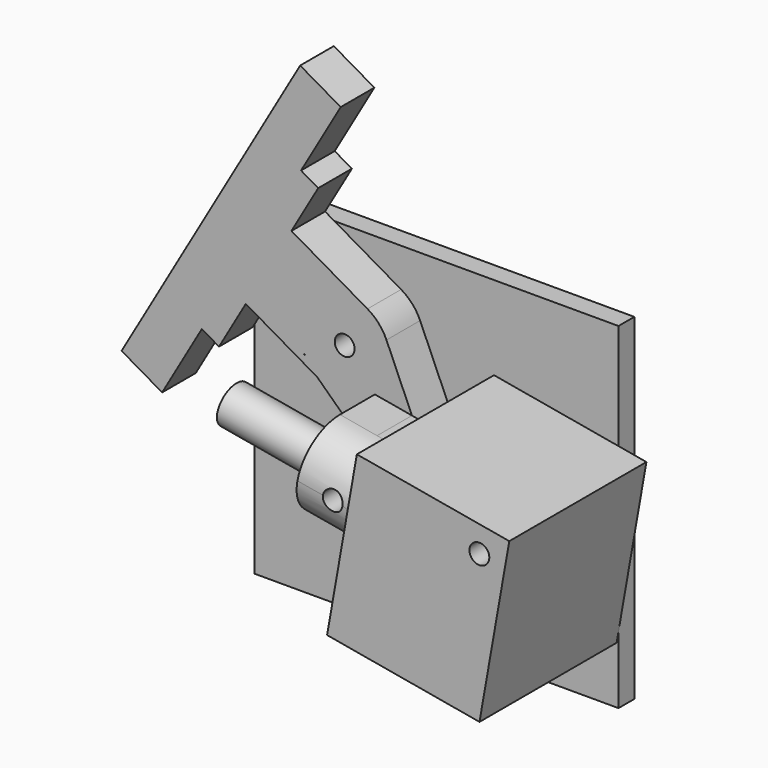
from build123d import *

# Parameters (mm, degrees)
F1_DEPTH    = 10.6
F2_DEPTH    = 43.2
F3_R        = 11
F4_DEPTH    = 2
F5_R        = 5
F6_DEPTH    = 43.4
F7_R        = 2.5
F8_DEPTH    = 22
F9_T1_DEPTH = 73
F9_T3_DEPTH = 73
F10_W       = 91.6676837951
F10_H       = 84.7782492638
F11_DEPTH   = 5
F12_R       = 2.5
F13_DEPTH   = 74.8
F15_DEPTH   = 10.6


# Not quite as in the source:
# - a fillet or chamfer that OpenCascade refuses, or shapes differently, is made with other operations: its cross-section is extruded or revolved along the edge and cut away or added
# - a feature of the source that left no trace in its solid (it failed there, or was rolled back) is left out
# - a feature names something its author has since deleted; it is built from what else it names


with BuildPart() as f1:
    # F0 (on Front) → F1 (new body)
    with BuildSketch(Plane.XZ):
        with BuildLine():
            Line((20.5230552312, -18.1992913043), (10.5343781692, 4.6126864827))
            ThreePointArc((10.5343781692, 4.6126864827), (0.6372216988, 11.4823320152), (-9.9592921435, 5.75))
            ThreePointArc((-9.9592921435, 5.75), (-11.496683076, 0.276185173), (-10.2239091523, -5.2651383312))
            Line((-10.2239091523, -5.2651383312), (-10.0330621935, -5.2987897992))
            Line((-10.0330621935, -5.2987897992), (-10.0760856471, -5.5427879295))
            ThreePointArc((-10.0760856471, -5.5427879295), (-9.1133059009, -7.0141040451), (-7.937476981, -8.3214457383))
            Line((-7.937476981, -8.3214457383), (0.0076867142, -15.9000031098))
            ThreePointArc((0.0076867142, -15.9000031098), (4.1721880916, -16.865197921), (7.4918654025, -19.5586001001))
            Line((7.4918654025, -19.5586001001), (12.1068221008, -20.3723414808))
            ThreePointArc((12.1068221008, -20.3723414808), (14.7867308402, -18.3159751797), (17.0688414833, -20.8064619249))
            ThreePointArc((17.0688414833, -20.8064619249), (17.0593282285, -21.0243512818), (17.0308608658, -21.2405823691))
            Line((17.0308608658, -21.2405823691), (20.9700918779, -21.9351750798))
            ThreePointArc((20.9700918779, -21.9351750798), (21.0227999926, -20.0341798777), (20.5230552312, -18.1992913043))
        make_face()
        with BuildLine():
            ThreePointArc((2.5, 0), (-0.6470476128, -2.4148145657), (-2.1650635095, 1.25))
            ThreePointArc((-2.1650635095, 1.25), (0.6470476128, 2.4148145657), (2.5, 0))
        make_face(mode=Mode.SUBTRACT)
        with BuildLine():
            ThreePointArc((10.0824414506, -25.509887777), (16.5964769767, -26.9821152755), (20.9700918779, -21.9351750798))
            Line((20.9700918779, -21.9351750798), (17.0308608658, -21.2405823691))
            ThreePointArc((17.0308608658, -21.2405823691), (14.1347210391, -23.2684813075), (12.1068221008, -20.3723414808))
            Line((12.1068221008, -20.3723414808), (7.4918654025, -19.5586001001))
            ThreePointArc((7.4918654025, -19.5586001001), (8.9071937501, -22.0966835606), (9.4890434601, -24.9438704))
            Line((9.4890434601, -24.9438704), (10.0824414506, -25.509887777))
        make_face()
        with BuildLine():
            Line((3.0158426859, -18.7693565289), (9.4890434601, -24.9438704))
            ThreePointArc((9.4890434601, -24.9438704), (8.9071937501, -22.0966835606), (7.4918654025, -19.5586001001))
            Line((7.4918654025, -19.5586001001), (3.0158426859, -18.7693565289))
        make_face()
        with BuildLine():
            ThreePointArc((7.4918654025, -19.5586001001), (4.1721880916, -16.865197921), (0.0076867142, -15.9000031098))
            Line((0.0076867142, -15.9000031098), (3.0158426859, -18.7693565289))
            Line((3.0158426859, -18.7693565289), (7.4918654025, -19.5586001001))
        make_face()
    extrude(amount=F1_DEPTH)

    # F14 (on face) → F15 (join)
    with BuildSketch(Plane.XZ.offset(10.6)):
        with BuildLine():
            Line((-31.664557856, -10.5859724576), (-24.914557856, 1.1053704935))
            Line((-24.914557856, 1.1053704935), (-6.941731015, -9.2712459212))
            Line((-6.941731015, -9.2712459212), (-7.937476981, -8.3214457383))
            ThreePointArc((-7.937476981, -8.3214457383), (-9.1133059009, -7.0141040451), (-10.0760856471, -5.5427879295))
            ThreePointArc((-10.0760856471, -5.5427879295), (-10.1509467311, -5.4044685642), (-10.2239091523, -5.2651383312))
            ThreePointArc((-10.2239091523, -5.2651383312), (-11.496683076, 0.276185173), (-9.9592921435, 5.75))
            Line((-9.9592921435, 5.75), (-23.4946848749, 13.564662637))
            Line((-23.4946848749, 13.564662637), (-35.9946848749, -8.0859724576))
            Line((-35.9946848749, -8.0859724576), (-31.664557856, -10.5859724576))
        make_face()
        with BuildLine():
            Line((-17.7446848749, 23.5239547806), (-23.4946848749, 13.564662637))
            Line((-23.4946848749, 13.564662637), (-9.9592921435, 5.75))
            ThreePointArc((-9.9592921435, 5.75), (-2.9764190187, 11.1081470023), (5.75, 9.9592921435))
            Line((5.75, 9.9592921435), (-13.414557856, 21.0239547806))
            Line((-13.414557856, 21.0239547806), (-6.664557856, 32.7152977317))
            Line((-6.664557856, 32.7152977317), (-10.9946848749, 35.2152977317))
            Line((-10.9946848749, 35.2152977317), (-17.7446848749, 23.5239547806))
        make_face()
        Polygon((-41.6238499995, -4.8359724576), (-35.9946848749, -8.0859724576), (-23.4946848749, 13.564662637), (-17.7446848749, 23.5239547806), (-10.9946848749, 35.2152977317), (-16.6238499995, 38.4652977317), align=None)
        Polygon((-45.9946848749, -25.4064805333), (-35.9946848749, -8.0859724576), (-41.6238499995, -4.8359724576), (-16.6238499995, 38.4652977317), (-10.9946848749, 35.2152977317), (-0.9946848749, 52.5358058073), (-11.2137846395, 58.4358058073), (-56.2137846395, -19.5064805333), align=None)
    extrude(amount=-F15_DEPTH)


with BuildPart() as f2:
    # F0 (on Front) → F2 (new body)
    with BuildSketch(Plane.XZ):
        Polygon((29.1525274041, -1.4447444142), (25.4017267665, -22.7165918793), (21.6509261288, -43.9884393443), (60.0584284963, -50.7607182734), (67.5600297715, -8.2170233432), align=None)
    extrude(amount=F2_DEPTH)

    # F3 (on face) → F4 (join)
    with BuildSketch(Plane(origin=(28.5205369873, 0, -5.0289401751), x_dir=(0, -1, 0), z_dir=(-0.984807753, 0, 0.1736481777))):
        with Locations((21.6, -17.9605122421)):
            Circle(F3_R)
    extrude(amount=F4_DEPTH)

    # F5 (on face) → F6 (join)
    with BuildSketch(Plane(origin=(26.5509214812, 0, -4.6816438198), x_dir=(0, -1, 0), z_dir=(-0.984807753, 0, 0.1736481777))):
        with Locations((21.6, -17.9605122421)):
            Circle(F5_R)
    extrude(amount=F6_DEPTH)


with BuildPart() as f8:
    # F7 (on face) → F8 (new body)
    with BuildSketch(Plane.XZ.offset(10.6)):
        with BuildLine():
            Line((3.7954417519, -30.0765136091), (21.5219813061, -33.2021808071))
            Line((21.5219813061, -33.2021808071), (25.3422412148, -11.5364102408))
            Line((25.3422412148, -11.5364102408), (16.9582685695, -10.0580896579))
            Line((16.9582685695, -10.0580896579), (20.5230552312, -18.1992913043))
            ThreePointArc((20.5230552312, -18.1992913043), (18.2970883196, -26.1309502128), (10.0824414506, -25.509887777))
            Line((10.0824414506, -25.509887777), (5.3899032629, -21.0338730293))
            Line((5.3899032629, -21.0338730293), (3.7954417519, -30.0765136091))
        make_face()
        with BuildLine():
            Line((20.5230552312, -18.1992913043), (16.9582685695, -10.0580896579))
            Line((16.9582685695, -10.0580896579), (7.6157016605, -8.4107430428))
            Line((7.6157016605, -8.4107430428), (5.3899032629, -21.0338730293))
            Line((5.3899032629, -21.0338730293), (10.0824414506, -25.509887777))
            ThreePointArc((10.0824414506, -25.509887777), (18.2970883196, -26.1309502128), (20.5230552312, -18.1992913043))
        make_face()
        with Locations((14.5688414833, -20.8064619249)):
            Circle(F7_R, mode=Mode.SUBTRACT)
    extrude(amount=F8_DEPTH)

    # F9: fillet of radius 11 on 2 edges, made by hand

    # F9_s2 → F9_t1 (cut)
    with BuildSketch(Plane(origin=(53.6331346891, 0, -9.4569687057), x_dir=(0, 1, 0), z_dir=(-0.984807753, 0, 0.1736481777))):
        with BuildLine():
            ThreePointArc((-21.6, 6.9605122421), (-29.3781745931, 10.1823376491), (-32.6, 17.9605122421))
            Line((-32.6, 17.9605122421), (-32.6, 6.9605122421))
            Line((-32.6, 6.9605122421), (-21.6, 6.9605122421))
        make_face()
    extrude(amount=F9_T1_DEPTH, mode=Mode.SUBTRACT)

    # F9_s4 → F9_t3 (cut)
    with BuildSketch(Plane(origin=(-18.2578312808, 0, 3.219348264), x_dir=(0, 1, 0), z_dir=(0.984807753, 0, -0.1736481777))):
        with BuildLine():
            ThreePointArc((-21.6, -28.9605122421), (-29.3781745931, -25.7386868352), (-32.6, -17.9605122421))
            Line((-32.6, -17.9605122421), (-32.6, -28.9605122421))
            Line((-32.6, -28.9605122421), (-21.6, -28.9605122421))
        make_face()
    extrude(amount=F9_T3_DEPTH, mode=Mode.SUBTRACT)


with BuildPart() as f11:
    # F10 (on face) → F11 (new body)
    with BuildSketch(Plane.XZ):
        with Locations((14.6878799424, -22.7255448699)):
            Rectangle(F10_W, F10_H)
        with BuildLine():
            Line((10.5343781692, 4.6126864827), (20.5230552312, -18.1992913043))
            ThreePointArc((20.5230552312, -18.1992913043), (21.0227999926, -20.0341798777), (20.9700918779, -21.9351750798))
            Line((20.9700918779, -21.9351750798), (17.0308608658, -21.2405823691))
            ThreePointArc((17.0308608658, -21.2405823691), (17.0593282285, -21.0243512818), (17.0688414833, -20.8064619249))
            ThreePointArc((17.0688414833, -20.8064619249), (14.7867308402, -18.3159751797), (12.1068221008, -20.3723414808))
            Line((12.1068221008, -20.3723414808), (7.4918654025, -19.5586001001))
            ThreePointArc((7.4918654025, -19.5586001001), (4.1721880916, -16.865197921), (0.0076867142, -15.9000031098))
            Line((0.0076867142, -15.9000031098), (-7.937476981, -8.3214457383))
            ThreePointArc((-7.937476981, -8.3214457383), (-9.1133059009, -7.0141040451), (-10.0760856471, -5.5427879295))
            Line((-10.0760856471, -5.5427879295), (-10.0330621935, -5.2987897992))
            Line((-10.0330621935, -5.2987897992), (-10.2239091523, -5.2651383312))
            ThreePointArc((-10.2239091523, -5.2651383312), (-11.496683076, 0.276185173), (-9.9592921435, 5.75))
            ThreePointArc((-9.9592921435, 5.75), (0.6372216988, 11.4823320152), (10.5343781692, 4.6126864827))
        make_face(mode=Mode.SUBTRACT)
    extrude(amount=-F11_DEPTH)

    # F0 (on Front) → F11, piece 2 (join)
    with BuildSketch(Plane.XZ):
        with BuildLine():
            Line((20.5230552312, -18.1992913043), (10.5343781692, 4.6126864827))
            ThreePointArc((10.5343781692, 4.6126864827), (0.6372216988, 11.4823320152), (-9.9592921435, 5.75))
            ThreePointArc((-9.9592921435, 5.75), (-11.496683076, 0.276185173), (-10.2239091523, -5.2651383312))
            Line((-10.2239091523, -5.2651383312), (-10.0330621935, -5.2987897992))
            Line((-10.0330621935, -5.2987897992), (-10.0760856471, -5.5427879295))
            ThreePointArc((-10.0760856471, -5.5427879295), (-9.1133059009, -7.0141040451), (-7.937476981, -8.3214457383))
            Line((-7.937476981, -8.3214457383), (0.0076867142, -15.9000031098))
            ThreePointArc((0.0076867142, -15.9000031098), (4.1721880916, -16.865197921), (7.4918654025, -19.5586001001))
            Line((7.4918654025, -19.5586001001), (12.1068221008, -20.3723414808))
            ThreePointArc((12.1068221008, -20.3723414808), (14.7867308402, -18.3159751797), (17.0688414833, -20.8064619249))
            ThreePointArc((17.0688414833, -20.8064619249), (17.0593282285, -21.0243512818), (17.0308608658, -21.2405823691))
            Line((17.0308608658, -21.2405823691), (20.9700918779, -21.9351750798))
            ThreePointArc((20.9700918779, -21.9351750798), (21.0227999926, -20.0341798777), (20.5230552312, -18.1992913043))
        make_face()
        with BuildLine():
            ThreePointArc((2.5, 0), (-0.6470476128, -2.4148145657), (-2.1650635095, 1.25))
            ThreePointArc((-2.1650635095, 1.25), (0.6470476128, 2.4148145657), (2.5, 0))
        make_face(mode=Mode.SUBTRACT)
        with BuildLine():
            ThreePointArc((12.1068221008, -20.3723414808), (14.1347210391, -23.2684813075), (17.0308608658, -21.2405823691))
            Line((17.0308608658, -21.2405823691), (12.1068221008, -20.3723414808))
        make_face()
        with BuildLine():
            Line((12.1068221008, -20.3723414808), (17.0308608658, -21.2405823691))
            ThreePointArc((17.0308608658, -21.2405823691), (17.0593282285, -21.0243512818), (17.0688414833, -20.8064619249))
            ThreePointArc((17.0688414833, -20.8064619249), (14.7867308402, -18.3159751797), (12.1068221008, -20.3723414808))
        make_face()
    extrude(amount=-F11_DEPTH)


with BuildPart() as f13_tool:
    # F12 (on face) → F13 (new body)
    with BuildSketch(Plane.XZ.offset(43.2)):
        with Locations((60.0300662221, -13.489560583)):
            Circle(F12_R)
    extrude(amount=-F13_DEPTH)


with BuildPart() as f2_1:
    add(f2.part)

    # F13: cut by f13_tool
    add(f13_tool.part, mode=Mode.SUBTRACT)


with BuildPart() as f11_1:
    add(f11.part)

    # F13: cut by f13_tool
    add(f13_tool.part, mode=Mode.SUBTRACT)


solid = Compound([f1.part, f8.part, f2_1.part, f11_1.part])
